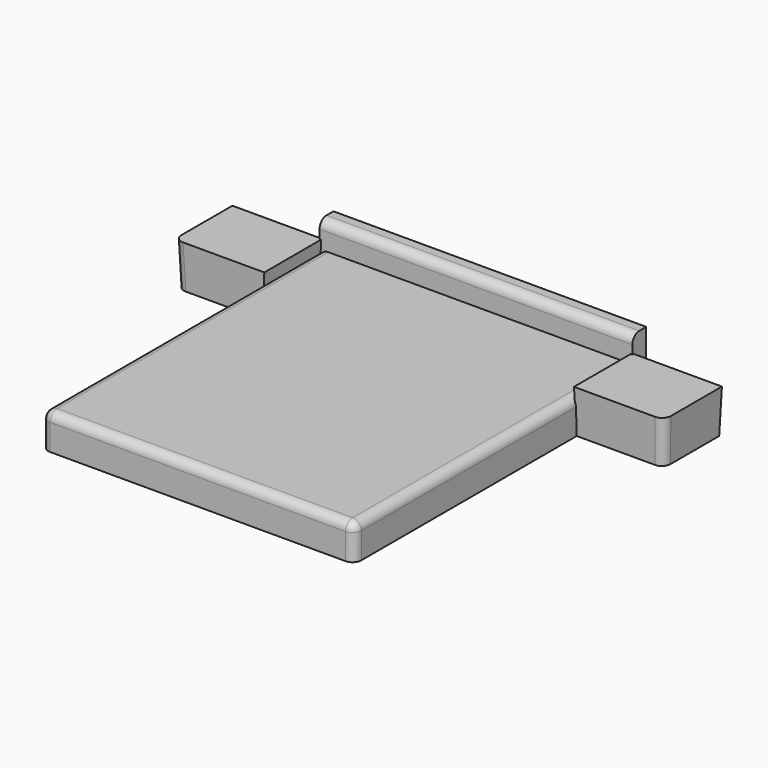
from build123d import *

# Parameters (mm, degrees)
F0_W                     = 36
F0_H                     = 2
F1_DEPTH                 = 7
F2_DEPTH                 = 4
F0_W_2                   = 10
F0_H_2                   = 8
F3_DEPTH                 = 5
DRAFT_F3_DRAFTED_ANGLE   = -2
DRAFT_F3_2_DRAFTED_ANGLE = -2
F4_R                     = 1


# Not quite as in the source:
# - an extrude with a draft is written as a straight extrude whose walls are then drafted


with BuildPart() as f1:
    # F0 (on Top) → F1 (new body)
    with BuildSketch(Plane.XY):
        with Locations((18, 1)):
            Rectangle(F0_W, F0_H)
    extrude(amount=F1_DEPTH)

    # F0 (on Top) → F2 (join)
    with BuildSketch(Plane.XY):
        Polygon((0, -8), (0, -40), (36, -40), (36, -8), (36, 0), (0, 0), align=None)
    extrude(amount=F2_DEPTH)


with BuildPart() as f3_drafted:
    # F0 (on Top) → F3 (new body)
    with BuildSketch(Plane.XY):
        with Locations((-5, -4)):
            Rectangle(F0_W_2, F0_H_2)
    extrude(amount=F3_DEPTH)

    # draft_F3_drafted
    draft_f3_drafted_walls = [f3_drafted.faces().sort_by_distance(p)[0] for p in [
        (-5, -8, 3.3333333333),
        (0, -4, 3.3333333333),
        (-5, 0, 3.3333333333),
        (-10, -4, 3.3333333333),
    ]]
    draft(draft_f3_drafted_walls, neutral_plane=Plane.XY, angle=DRAFT_F3_DRAFTED_ANGLE)


with BuildPart() as f1_1:
    add(f1.part)

    # join_F3_drafted: union F3_drafted
    add(f3_drafted.part)


with BuildPart() as f3_2_drafted:
    # F0 (on Top) → F3, piece 2 (new body)
    with BuildSketch(Plane.XY):
        with Locations((41, -4)):
            Rectangle(F0_W_2, F0_H_2)
    extrude(amount=F3_DEPTH)

    # draft_F3_2_drafted
    draft_f3_2_drafted_walls = [f3_2_drafted.faces().sort_by_distance(p)[0] for p in [
        (36, -4, 3.3333333333),
        (41, -8, 3.3333333333),
        (46, -4, 3.3333333333),
        (41, 0, 3.3333333333),
    ]]
    draft(draft_f3_2_drafted_walls, neutral_plane=Plane.XY, angle=DRAFT_F3_2_DRAFTED_ANGLE)


with BuildPart() as f1_2:
    add(f1_1.part)

    # join_F3_2_drafted: union F3_2_drafted
    add(f3_2_drafted.part)

    # F4
    f4_edges = [f1_2.edges().sort_by_distance(p)[0] for p in [
        (18, 0, 7),
        (36, -40, 2),
        (0, -40, 2),
        (18, -40, 4),
        (36, -24.069842, 4),
        (0, -24.069842, 4),
        (-10.087302, -8.087302, 2.5),
        (46.087302, -8.087302, 2.5),
    ]]
    fillet(f4_edges, radius=F4_R)


solid = f1_2.part
